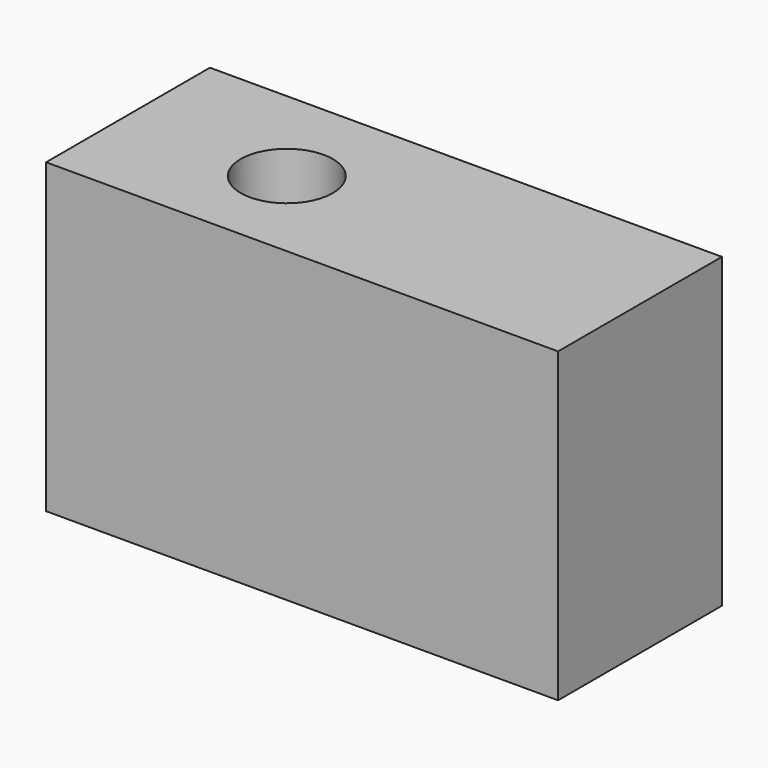
from build123d import *

# Parameters (mm, degrees)
F0_W     = 25
F0_H     = 10
F1_DEPTH = 15
F3_D     = 4.5
F3_DEPTH = 14.2
F3_TIP   = 1.3519363928


with BuildPart() as f1:
    # F0 (on Top) → F1 (new body)
    with BuildSketch(Plane.XY):
        with Locations((-34.2963750242, -4.0348231601)):
            Rectangle(F0_W, F0_H)
    extrude(amount=F1_DEPTH)

    # F3
    with Locations(Plane.XY.offset(15)):
        with Locations((-38.9182306826, -4.1914577596)):
            Hole(F3_D / 2, depth=F3_DEPTH)
            with Locations((0, 0, -(F3_DEPTH + F3_TIP / 2))):  # 118° drill point
                Cone(0, F3_D / 2, F3_TIP, mode=Mode.SUBTRACT)


solid = f1.part
